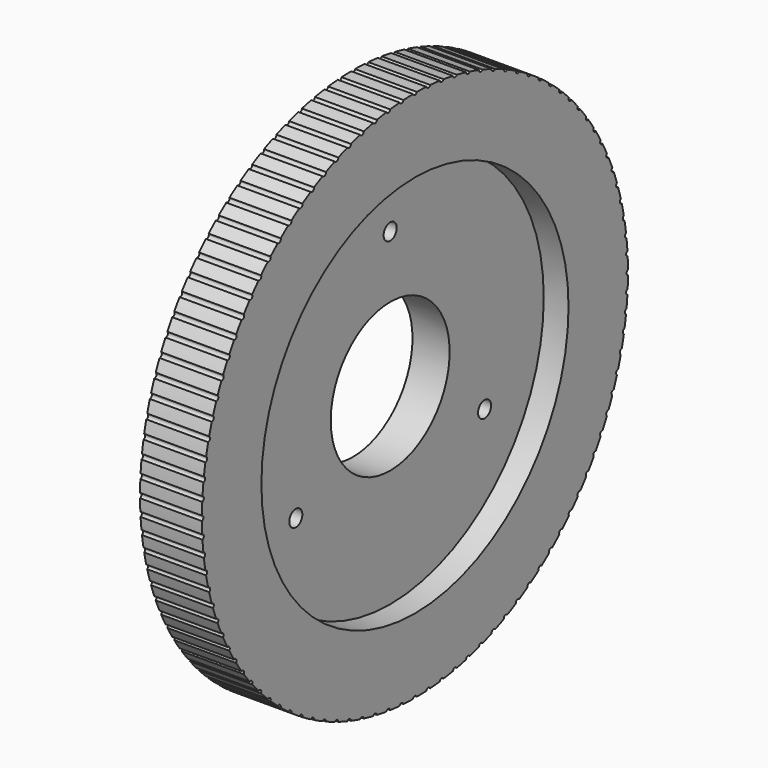
from build123d import *

# Parameters (mm, degrees)
F0_R            = 107.5
F1_DEPTH        = 25
F2_R            = 77.5
F3_DEPTH        = 10
F5_D            = 6.6
F5_CSINK_D      = 13.44
F5_CSINK_ANGLE  = 90
F6_R            = 30
F7_DEPTH        = 25
F9_DEPTH        = 25
F9_COPIES_COUNT = 100


# Not quite as in the source:
# - a pattern or mirror of a feature is missing from the dataset's text; its kind, count and spacing are read off the source's solid


with BuildPart() as f1:
    # F0 (on Right) → F1 (new body)
    with BuildSketch(Plane.YZ):
        Circle(F0_R)
    extrude(amount=F1_DEPTH)

    # F2 (on face) → F3 (cut)
    with BuildSketch(Plane.YZ.offset(25)):
        Circle(F2_R)
    extrude(amount=-F3_DEPTH, mode=Mode.SUBTRACT)

    # F5 (through all)
    with Locations(Plane(origin=(0, 0, 0), x_dir=(0, -1, 0), z_dir=(-1, 0, 0))):
        with Locations((0, 55), (47.6313972081, -27.5), (-47.6313972081, -27.5)):
            CounterSinkHole(F5_D / 2, F5_CSINK_D / 2, counter_sink_angle=F5_CSINK_ANGLE)

    # F6 (on face) → F7 (cut)
    with BuildSketch(Plane(origin=(0, 0, 0), x_dir=(0, -1, 0), z_dir=(-1, 0, 0))):
        Circle(F6_R)
    extrude(amount=-F7_DEPTH, mode=Mode.SUBTRACT)

    # F8 (on face) → F9 (cut)
    with BuildSketch(Plane(origin=(0, 0, 0), x_dir=(0, -1, 0), z_dir=(-1, 0, 0))):
        with BuildLine():
            ThreePointArc((-0.9613668942, 107.495701187), (0, 106.7762187272), (0.9613668942, 107.495701187))
            ThreePointArc((0.9613668942, 107.495701187), (0, 107.5), (-0.9613668942, 107.495701187))
        make_face()
    f9 = extrude(amount=-F9_DEPTH, mode=Mode.SUBTRACT)

    # F9_copies: F9 ×100 about axis
    f9_copies_axis = Axis((0, 0, 0), (1, 0, 0))
    for i in range(1, F9_COPIES_COUNT):
        add(f9.rotate(f9_copies_axis, i * 360 / F9_COPIES_COUNT), mode=Mode.SUBTRACT)


solid = f1.part
